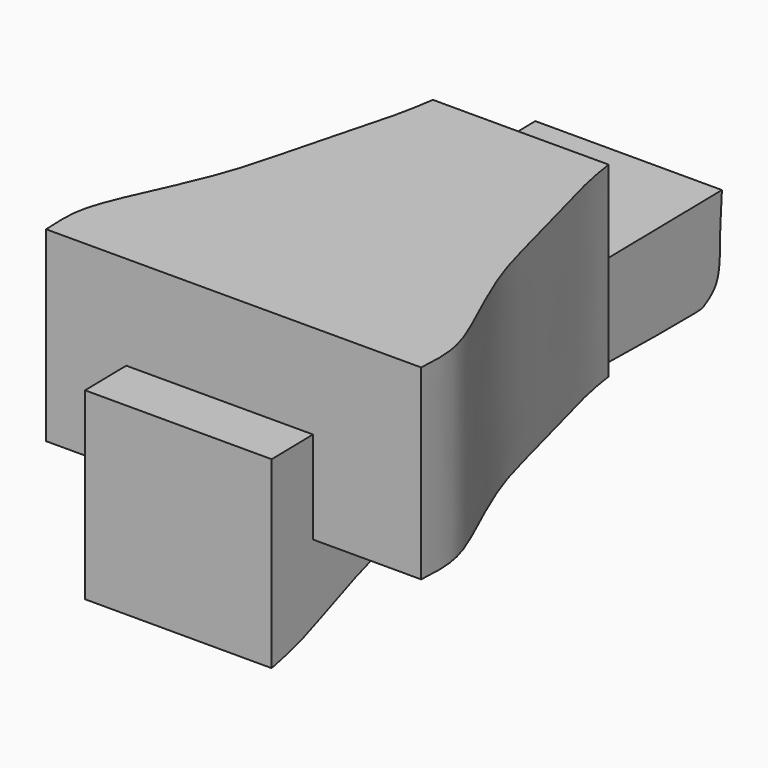
from build123d import *

# Parameters (mm, degrees)
F2_DEPTH = 25
F3_DEPTH = 25
F4_ANGLE = -90


# Not quite as in the source:
# - a feature of the source that left no trace in its solid (it failed there, or was rolled back) is left out


with BuildPart() as f2:
    # F0 (on Top) → F2 (new body)
    with BuildSketch(Plane.XY):
        with BuildLine():
            add(Edge.make_bspline(
                [(-27.228333056, -3.449567128), (-27.3434241217, -1.6475910188), (-27.5953592018, 2.2530633156), (-24.5578786757, 9.1739413778), (-20.1021081789, 18.7662622294), (-18.0224229491, 28.2501608363), (-14.6119129517, 39.9429075555), (-14.1578250024, 43.3578089685), (-13.9501262456, 44.7319447994)],
                knots=[0, 0, 0, 0, 0.1366154369, 0.2958664845, 0.4845995186, 0.6720222775, 0.8738533997, 1, 1, 1, 1], degree=3))
            Line((-27.228333056, -3.449567128), (22.9792274906, -3.3865838763))
            add(Edge.make_bspline(
                [(22.9792274906, -3.3865838763), (23.0897971962, -1.5843246853), (23.3319450885, 2.3169494552), (20.2771102546, 9.2301849667), (15.7972875015, 18.8112964961), (13.6938145588, 28.2899475088), (10.2539792336, 39.9741007608), (9.7913250294, 43.3878521598), (9.5801793417, 44.7614625681)],
                knots=[0, 0, 0, 0, 0.1366154369, 0.2958664845, 0.4845995186, 0.6720222775, 0.8738533997, 1, 1, 1, 1], degree=3))
            Line((9.5801793417, 44.7614625681), (-2.1849549375, 44.7319447994))
            Line((-2.1849549375, 44.7319447994), (-13.9501262456, 44.7319447994))
        make_face()
    extrude(amount=F2_DEPTH)


with BuildPart() as f3:
    # F1 (on Right) → F3 (new body)
    with BuildSketch(Plane.YZ):
        with BuildLine():
            Line((16.9688649476, -12.1081583202), (-7.6804482378, -12.1081583202))
            add(Edge.make_bspline(
                [(-7.6804482378, -12.1081583202), (-7.3344915169, -13.7336139495), (-6.4358902415, -17.9556348362), (-0.4236596256, -29.8799173597), (3.3012366068, -49.4373461154), (2.4811298634, -54.1997913125), (5.8307967283, -58.1268067059), (5.6143806257, -59.1152093352), (5.1285618546, -83.8034786686), (5.6091659498, -84.5053082309), (7.1854008957, -87.2927879477), (12.7938111558, -87.1166442137), (16.2991404351, -87.3850513493), (18.0650819093, -87.5202715397)],
                knots=[0, 0, 0, 0, 0.0827675381, 0.2149835826, 0.3724587977, 0.449999816, 0.5217745436, 0.5670647447, 0.740339061, 0.7800065219, 0.8353564944, 0.9170546411, 1, 1, 1, 1], degree=3))
            Line((18.0650819093, -87.5202715397), (16.9688649476, -12.1081583202))
        make_face()
    extrude(amount=F3_DEPTH)


with BuildPart() as f3_1:
    # F4: moved
    add(f3.part.rotate(Axis((12.5, 16.9688649476, -12.1081583202), (-1, 0, 0)), F4_ANGLE))


with BuildPart() as f2_1:
    # F5: moved
    add(f2.part.moved(Location((16.5, 27.3, -24.4))))


solid = Compound([f3_1.part, f2_1.part])
